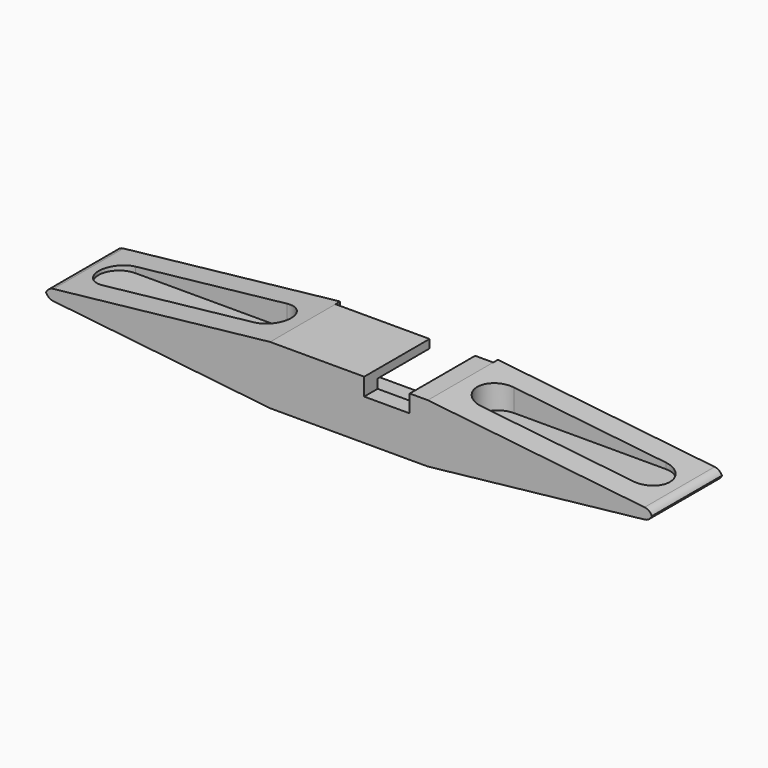
from build123d import *

# Parameters (mm, degrees)
F1_DEPTH      = 19.05
F4_DEPTH      = 11.43
F8_W          = 58.2950823009
F8_H          = 18.0758163333
F9_DEPTH      = 19.051
F9_DEPTH_BACK = 11.74174
F11_W         = 68.613074236
F11_H         = 25.4
F12_DEPTH     = 2.54
F13_W         = 19.8203250766
F13_H         = 44.8987269774
F14_DEPTH     = 7.62


with BuildPart() as f1:
    # F0 (on Front) → F1 (new body, symmetric)
    with BuildSketch(Plane.XZ):
        with BuildLine():
            Line((16.493462882, 12.7), (-77.7931159433, 2.3487282923))
            ThreePointArc((-77.7931159433, 2.3487282923), (-79.6990393329, 1.6031312535), (-80.9712142796, 0))
            Line((-80.9712142796, 0), (50.8, 0))
            Line((50.8, 0), (50.8, 12.7))
            Line((50.8, 12.7), (16.493462882, 12.7))
        make_face()
    extrude(amount=F1_DEPTH, both=True)

    # F3 (on offset) → F4 (cut)
    with BuildSketch(Plane.XY.offset(12.7)):
        with BuildLine():
            Line((-64.5951760395, -8.7044802925), (1.4448239605, -8.7044802925))
            ThreePointArc((1.4448239605, -8.7044802925), (10.3064292543, 0.1571250013), (1.4448239605, 9.0187302952))
            Line((1.4448239605, 9.0187302952), (-64.5951760395, 9.0187302952))
            ThreePointArc((-64.5951760395, 9.0187302952), (-73.4567813333, 0.1571250013), (-64.5951760395, -8.7044802925))
        make_face()
    extrude(amount=-F4_DEPTH, mode=Mode.SUBTRACT)

    # F5: F1 across plane


with BuildPart() as f1_1:
    add(f1.part)
    add(f1.part.mirror(Plane.XY))

    # F7: F1 across plane


with BuildPart() as f1_2:
    add(f1_1.part)
    add(f1_1.part.mirror(Plane.YZ.offset(50.8)))

    # F8 (on Front) → F9 (cut, two sides)
    with BuildSketch(Plane.XZ) as f9_sk:
        with Locations((50.8, 0)):
            Rectangle(F8_W, F8_H)
    extrude(amount=-F9_DEPTH, mode=Mode.SUBTRACT)
    extrude(f9_sk.sketch, amount=F9_DEPTH_BACK, mode=Mode.SUBTRACT)

    # F11 (on offset) → F12 (cut)
    with BuildSketch(Plane.XZ.offset(-19.05)):
        with Locations((50.8, 0)):
            Rectangle(F11_W, F11_H)
    extrude(amount=F12_DEPTH, mode=Mode.SUBTRACT)

    # F13 (on offset) → F14 (cut)
    with BuildSketch(Plane.XY.offset(12.7)):
        with Locations((67.3308186233, -3.4829550423)):
            Rectangle(F13_W, F13_H)
    extrude(amount=-F14_DEPTH, mode=Mode.SUBTRACT)


solid = f1_2.part
